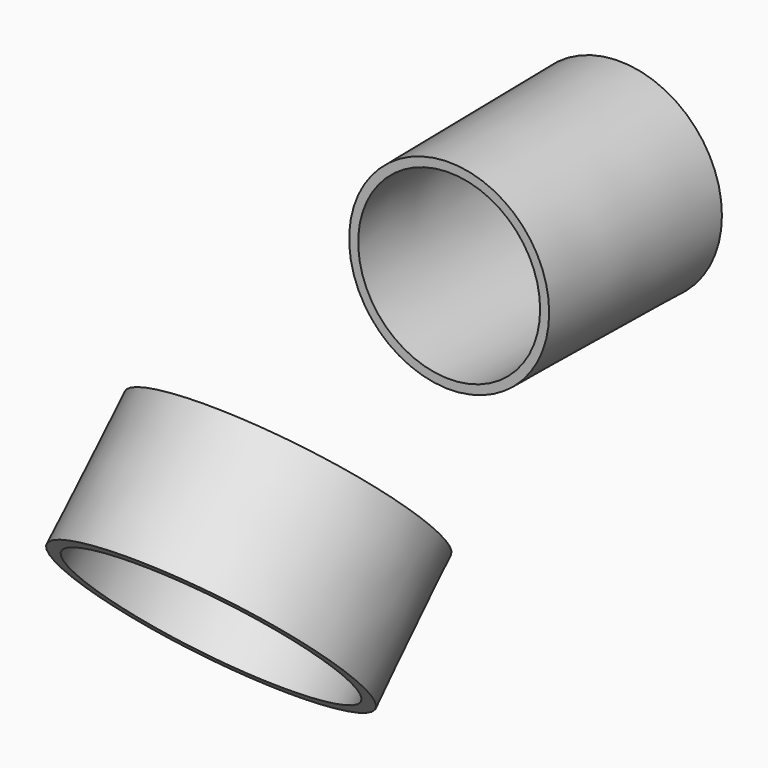
from build123d import *

# Parameters (mm, degrees)
F0_R     = 22.1
F1_DEPTH = 47
F1_TAPER = -0.7
F2_T     = -2
F3_R     = 31.5
F4_DEPTH = 30
F4_TAPER = -0.5
F5_T     = -2.8
F7_ANGLE = 45


# Not quite as in the source:
# - the program builds the solid bodies; features that only make, move or delete a surface that nothing else refers to are left out


with BuildPart() as f1:
    # F0 (on Front) → F1 (new body)
    with BuildSketch(Plane.XZ):
        Circle(F0_R)
    extrude(amount=-F1_DEPTH, taper=F1_TAPER)

    # F2
    f2_openings = [f1.faces().sort_by_distance(p)[0] for p in [
        (0, 47, 0),
        (0, 0, 0),
    ]]
    offset(amount=F2_T, openings=f2_openings, kind=Kind.INTERSECTION)


with BuildPart() as f4:
    # F3 (on Front) → F4 (new body)
    with BuildSketch(Plane.XZ):
        Circle(F3_R)
    extrude(amount=F4_DEPTH, taper=F4_TAPER)

    # F5
    f5_openings = [f4.faces().sort_by_distance(p)[0] for p in [
        (0, -30, 0),
        (0, 0, 0),
    ]]
    offset(amount=F5_T, openings=f5_openings, kind=Kind.INTERSECTION)


with BuildPart() as f4_1:
    # F7: moved
    add(f4.part.rotate(Axis((0, 0, 0), (1, 0, 0)), F7_ANGLE))


with BuildPart() as f4_2:
    # F8: moved
    add(f4_1.part.moved(Location((0, -44.5524342358, -20.2464051545))))


solid = Compound([f1.part, f4_2.part])
